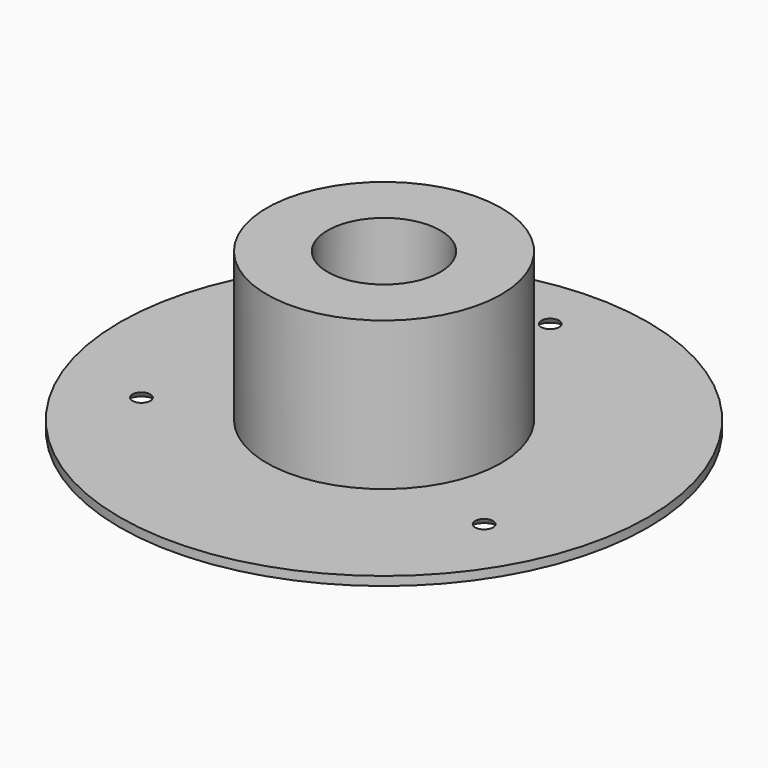
from build123d import *

# Parameters (mm, degrees)
F0_R     = 89
F0_R_2   = 3
F0_R_3   = 19
F1_DEPTH = 3
F2_R     = 39.5
F2_R_2   = 19
F3_DEPTH = 50


# Not quite as in the source:
# - a fillet or chamfer that OpenCascade refuses, or shapes differently, is made with other operations: its cross-section is extruded or revolved along the edge and cut away or added


with BuildPart() as f1:
    # F0 (on Top) → F1 (new body)
    with BuildSketch(Plane.XY):
        Circle(F0_R)
        with Locations((-57.735026919, -30)):
            Circle(F0_R_2, mode=Mode.SUBTRACT)
        with Locations((57.735026919, -30)):
            Circle(F0_R_2, mode=Mode.SUBTRACT)
        Circle(F0_R_3, mode=Mode.SUBTRACT)
        with Locations((0, 70)):
            Circle(F0_R_2, mode=Mode.SUBTRACT)
    extrude(amount=F1_DEPTH)

    # F2 (on face) → F3 (join)
    with BuildSketch(Plane.XY.offset(3)):
        Circle(F2_R)
        Circle(F2_R_2, mode=Mode.SUBTRACT)
    extrude(amount=F3_DEPTH)

    # F4: fillet of radius 5 on 3 edges, made by hand

    # F4_s1 → F4_t2 (revolve, cut)
    with BuildSketch(Plane.XZ.offset(30)):
        with BuildLine():
            ThreePointArc((60.735026919, 3), (62.5789898264, 0.8166998673), (65.3176026139, 0))
            Line((65.3176026139, 0), (60.735026919, 0))
            Line((60.735026919, 0), (60.735026919, 3))
        make_face()
    revolve(axis=Axis((57.735026919, -30, 0), (0, 0, 1)), mode=Mode.SUBTRACT)

    # F4_s3 → F4_t4 (revolve, cut)
    with BuildSketch(Plane.XZ.offset(-70)):
        with BuildLine():
            ThreePointArc((3, 3), (4.8439629074, 0.8166998673), (7.582575695, 0))
            Line((7.582575695, 0), (3, 0))
            Line((3, 0), (3, 3))
        make_face()
    revolve(axis=Axis((0, 70, 0), (0, 0, 1)), mode=Mode.SUBTRACT)

    # F4_s5 → F4_t6 (revolve, cut)
    with BuildSketch(Plane.XZ.offset(30)):
        with BuildLine():
            ThreePointArc((-54.735026919, 3), (-52.8910640115, 0.8166998673), (-50.152451224, 0))
            Line((-50.152451224, 0), (-54.735026919, 0))
            Line((-54.735026919, 0), (-54.735026919, 3))
        make_face()
    revolve(axis=Axis((-57.735026919, -30, 0), (0, 0, 1)), mode=Mode.SUBTRACT)


solid = f1.part
